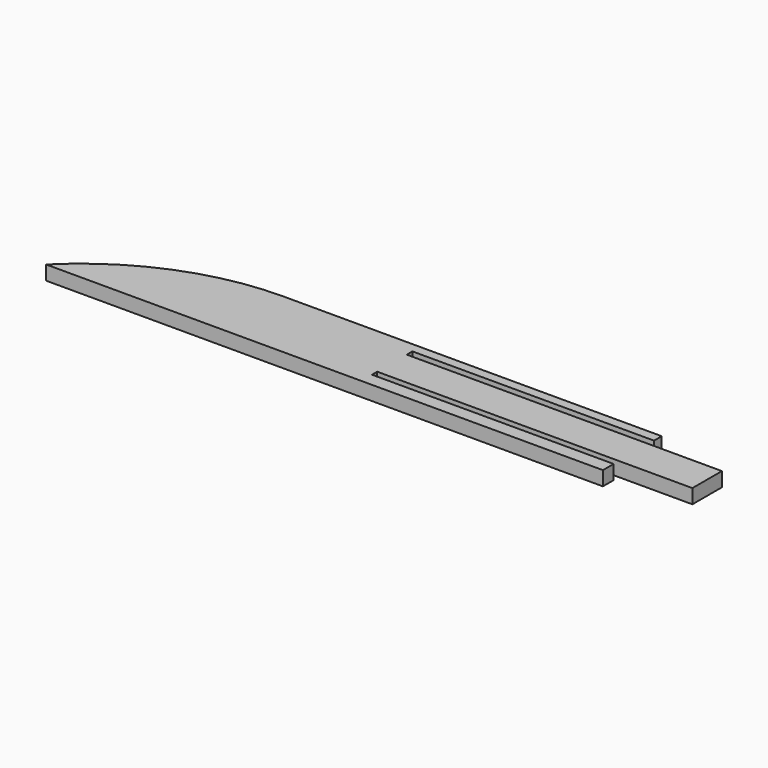
from build123d import *

# Parameters (mm, degrees)
F1_DEPTH    = 6
F2_DEPTH    = 0.8
F3_T1_DEPTH = 431.7925725323
F4_DEPTH    = 35


# Not quite as in the source:
# - a fillet or chamfer that OpenCascade refuses, or shapes differently, is made with other operations: its cross-section is extruded or revolved along the edge and cut away or added


with BuildPart() as f1:
    # F0 (on Top) → F1 (new body)
    with BuildSketch(Plane.XY):
        Polygon((150, 17.5), (-150, 17.5), (-150, -17.5), (150, -17.5), (150, -11.1123658717), (0, -11.1123658717), (0, -8.0123320222), (150, -8.0123320222), (150, 9.5545258373), (0, 9.5545258373), (0, 12.9128964618), (150, 12.9128964618), align=None)
    extrude(amount=F1_DEPTH)

    # F2 (add): faces of the model
    f2_faces = [f1.faces().sort_by_distance(p)[0] for p in [
        (-7.6230433236, -0.1272136786, 0),
        (-7.6230433236, -0.1272136786, 6),
    ]]
    extrude(f2_faces, amount=F2_DEPTH, dir=(0, 0, -1))

    # F3: fillet of radius 120.7106781187 on 1 edges, made by hand

    # F3_s2 → F3_t1 (cut)
    with BuildSketch(Plane.XY.offset(-213.2962862662)):
        with BuildLine():
            ThreePointArc((-65.0014854935, 17.5), (-110.9627394699, 8.4075593911), (-150, -17.5))
            Line((-150, -17.5), (-150, 17.5))
            Line((-150, 17.5), (-65.0014854935, 17.5))
        make_face()
    extrude(amount=F3_T1_DEPTH, mode=Mode.SUBTRACT)

    # F4 (cut): faces of the model
    f4_faces = [f1.faces().sort_by_distance(p)[0] for p in [
        (150, 15.2064482309, 2.6),
        (150, -14.3061829358, 2.6),
    ]]
    extrude(f4_faces, amount=-F4_DEPTH, mode=Mode.SUBTRACT)


solid = f1.part
